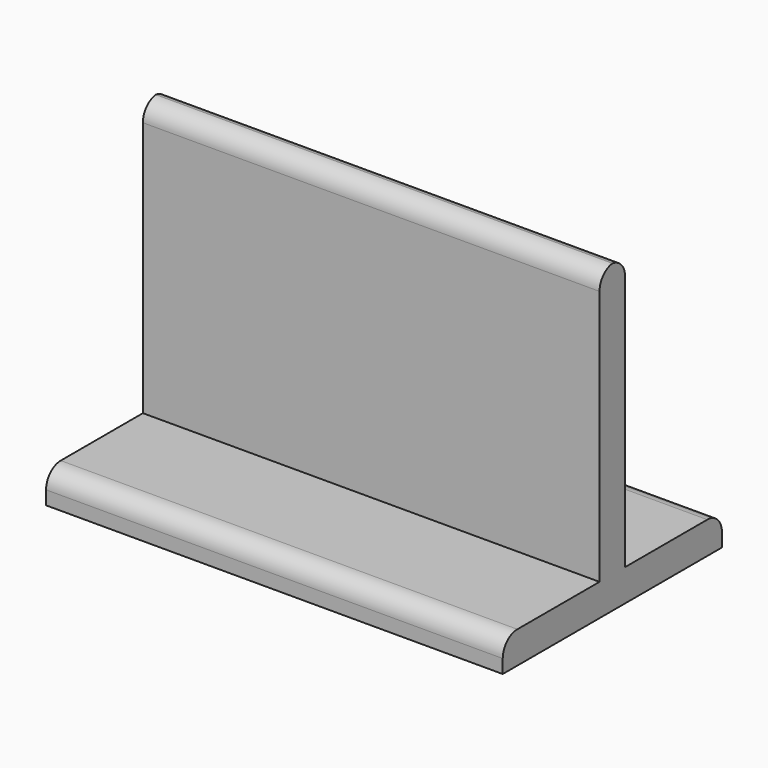
from build123d import *

# Parameters (mm, degrees)
F0_W        = 50
F0_H        = 30
F1_DEPTH    = 3.5
F2_R        = 2
F3_W        = 50
F3_H        = 3.5
F4_DEPTH    = 30
F5_T1_DEPTH = 60


# Not quite as in the source:
# - a fillet or chamfer that OpenCascade refuses, or shapes differently, is made with other operations: its cross-section is extruded or revolved along the edge and cut away or added


with BuildPart() as f1:
    # F0 (on Top) → F1 (new body)
    with BuildSketch(Plane.XY):
        Rectangle(F0_W, F0_H)
    extrude(amount=F1_DEPTH)

    # F2
    f2_edges = [f1.edges().sort_by_distance(p)[0] for p in [
        (0, 15, 3.5),
        (0, -15, 3.5),
    ]]
    fillet(f2_edges, radius=F2_R)

    # F3 (on face) → F4 (join)
    with BuildSketch(Plane.XY.offset(3.5)):
        Rectangle(F3_W, F3_H)
    extrude(amount=F4_DEPTH)

    # F5: fillet of radius 2 on 2 edges, made by hand

    # F5_s2 → F5_t1 (cut)
    with BuildSketch(Plane.YZ.offset(-30)):
        with BuildLine():
            ThreePointArc((-1.75, 31.5), (-1.1642135624, 32.9142135624), (0.25, 33.5))
            Line((0.25, 33.5), (-1.75, 33.5))
            Line((-1.75, 33.5), (-1.75, 31.5))
        make_face()
        with BuildLine():
            ThreePointArc((1.75, 31.5), (1.1642135624, 32.9142135624), (-0.25, 33.5))
            Line((-0.25, 33.5), (1.75, 33.5))
            Line((1.75, 33.5), (1.75, 31.5))
        make_face()
    extrude(amount=F5_T1_DEPTH, mode=Mode.SUBTRACT)


solid = f1.part
